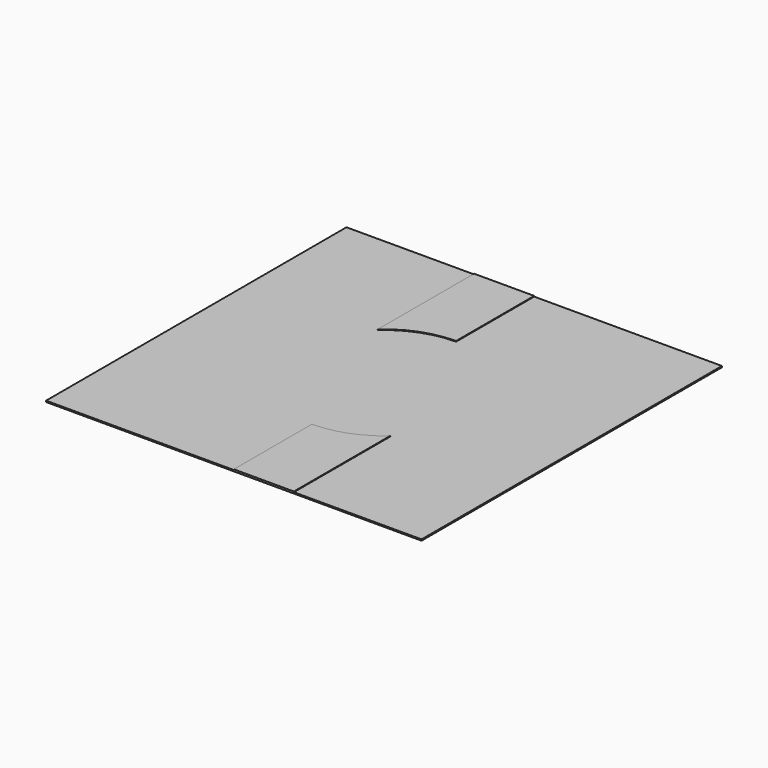
from build123d import *

# Parameters (mm, degrees)
F0_R     = 1790.7
F1_DEPTH = 25.4
F3_DEPTH = 25.4
F4_DEPTH = 25.4
F5_DEPTH = 38.1


# Not quite as in the source:
# - the program builds the solid bodies; features that only make, move or delete a surface that nothing else refers to are left out


with BuildPart() as f1:
    # F0 (on Top) → F1 (new body)
    with BuildSketch(Plane.XY):
        with BuildLine():
            Line((-1219.2, 3810.0001542995), (-3809.5957711624, 3810.0001542995))
            Line((-3809.5957711624, 3810.0001542995), (-3809.5957711624, -3809.9998457005))
            Line((-3809.5957711624, -3809.9998457005), (3.7253e-06, -3809.9998457005))
            Line((3.7253e-06, -3809.9998457005), (3.0473e-06, -3116.5800094754))
            Line((3.0473e-06, -3116.5800094754), (2.2873e-06, -2339.3399715424))
            Line((2.2873e-06, -2339.3399715424), (1.7881e-06, -1828.8))
            ThreePointArc((1.7881e-06, -1828.8), (-1708.414409752, -652.5562386122), (-1219.2, 1363.1070390839))
            Line((-1219.2, 1363.1070390839), (-1219.2, 2247.9000093898))
            Line((-1219.2, 2247.9000093898), (-1219.2, 3040.3800010681))
            Line((-1219.2, 3040.3800010681), (-1219.2, 3810.0001542995))
        make_face()
        with BuildLine():
            Line((3809.595778613, 3810.0001542995), (3.7253e-06, 3810.0001542995))
            Line((3.7253e-06, 3810.0001542995), (0, 3040.3800010681))
            Line((0, 3040.3800010681), (0, 2247.9000081977))
            Line((0, 2247.9000081977), (0, 1828.8))
            ThreePointArc((0, 1828.8), (1293.156881434, 1293.156881434), (1828.8, 0))
            ThreePointArc((1828.8, 0), (1669.4583559266, -746.6044721449), (1219.2000023767, -1363.1070369581))
            Line((1219.2000023767, -1363.1070369581), (1219.2000023767, -2339.3399703503))
            Line((1219.2000023767, -2339.3399703503), (1219.2000023767, -3116.5800082833))
            Line((1219.2000023767, -3116.5800082833), (1219.2000023767, -3809.9998457005))
            Line((1219.2000023767, -3809.9998457005), (3809.595778613, -3809.9998457005))
            Line((3809.595778613, -3809.9998457005), (3809.595778613, 3810.0001542995))
        make_face()
        with BuildLine():
            ThreePointArc((0, 1828.8), (-652.556237777, 1708.414410071), (-1219.2, 1363.1070390839))
            ThreePointArc((-1219.2, 1363.1070390839), (-1708.414409752, -652.5562386122), (1.7881e-06, -1828.8))
            ThreePointArc((1.7881e-06, -1828.8), (652.5562401017, -1708.4144091831), (1219.2000023767, -1363.1070369581))
            ThreePointArc((1219.2000023767, -1363.1070369581), (1669.4583559266, -746.6044721449), (1828.8, 0))
            ThreePointArc((1828.8, 0), (1293.156881434, 1293.156881434), (0, 1828.8))
        make_face()
        Circle(F0_R, mode=Mode.SUBTRACT)
    extrude(amount=F1_DEPTH)

    # F0 (on Top) → F3 (join)
    with BuildSketch(Plane.XY):
        with BuildLine():
            Line((-1219.2, 3810.0001542995), (-3809.5957711624, 3810.0001542995))
            Line((-3809.5957711624, 3810.0001542995), (-3809.5957711624, -3809.9998457005))
            Line((-3809.5957711624, -3809.9998457005), (3.7253e-06, -3809.9998457005))
            Line((3.7253e-06, -3809.9998457005), (3.0473e-06, -3116.5800094754))
            Line((3.0473e-06, -3116.5800094754), (2.2873e-06, -2339.3399715424))
            Line((2.2873e-06, -2339.3399715424), (1.7881e-06, -1828.8))
            ThreePointArc((1.7881e-06, -1828.8), (-1708.414409752, -652.5562386122), (-1219.2, 1363.1070390839))
            Line((-1219.2, 1363.1070390839), (-1219.2, 2247.9000093898))
            Line((-1219.2, 2247.9000093898), (-1219.2, 3040.3800010681))
            Line((-1219.2, 3040.3800010681), (-1219.2, 3810.0001542995))
        make_face()
        Polygon((3.7253e-06, 3810.0001542995), (-1219.2, 3810.0001542995), (-1219.2, 3040.3800010681), (0, 3040.3800010681), align=None)
        with BuildLine():
            Line((3809.595778613, 3810.0001542995), (3.7253e-06, 3810.0001542995))
            Line((3.7253e-06, 3810.0001542995), (0, 3040.3800010681))
            Line((0, 3040.3800010681), (0, 2247.9000081977))
            Line((0, 2247.9000081977), (0, 1828.8))
            ThreePointArc((0, 1828.8), (1293.156881434, 1293.156881434), (1828.8, 0))
            ThreePointArc((1828.8, 0), (1669.4583559266, -746.6044721449), (1219.2000023767, -1363.1070369581))
            Line((1219.2000023767, -1363.1070369581), (1219.2000023767, -2339.3399703503))
            Line((1219.2000023767, -2339.3399703503), (1219.2000023767, -3116.5800082833))
            Line((1219.2000023767, -3116.5800082833), (1219.2000023767, -3809.9998457005))
            Line((1219.2000023767, -3809.9998457005), (3809.595778613, -3809.9998457005))
            Line((3809.595778613, -3809.9998457005), (3809.595778613, 3810.0001542995))
        make_face()
        Polygon((3.0473e-06, -3116.5800094754), (3.7253e-06, -3809.9998457005), (1219.2000023767, -3809.9998457005), (1219.2000023767, -3116.5800082833), align=None)
    extrude(amount=F3_DEPTH)

    # F0 (on Top) → F4 (join)
    with BuildSketch(Plane.XY):
        Circle(F0_R)
    extrude(amount=F4_DEPTH)

    # F0 (on Top) → F5 (join)
    with BuildSketch(Plane.XY):
        Polygon((3.7253e-06, 3810.0001542995), (-1219.2, 3810.0001542995), (-1219.2, 3040.3800010681), (0, 3040.3800010681), align=None)
        with BuildLine():
            Line((0, 2247.9000081977), (-1219.2, 2247.9000093898))
            Line((-1219.2, 2247.9000093898), (-1219.2, 1363.1070390839))
            ThreePointArc((-1219.2, 1363.1070390839), (-652.556237777, 1708.414410071), (0, 1828.8))
            Line((0, 1828.8), (0, 2247.9000081977))
        make_face()
        Polygon((0, 3040.3800010681), (-1219.2, 3040.3800010681), (-1219.2, 2247.9000093898), (0, 2247.9000081977), align=None)
        with BuildLine():
            Line((1.7881e-06, -1828.8), (2.2873e-06, -2339.3399715424))
            Line((2.2873e-06, -2339.3399715424), (1219.2000023767, -2339.3399703503))
            Line((1219.2000023767, -2339.3399703503), (1219.2000023767, -1363.1070369581))
            ThreePointArc((1219.2000023767, -1363.1070369581), (652.5562401017, -1708.4144091831), (1.7881e-06, -1828.8))
        make_face()
        Polygon((2.2873e-06, -2339.3399715424), (3.0473e-06, -3116.5800094754), (1219.2000023767, -3116.5800082833), (1219.2000023767, -2339.3399703503), align=None)
        Polygon((3.0473e-06, -3116.5800094754), (3.7253e-06, -3809.9998457005), (1219.2000023767, -3809.9998457005), (1219.2000023767, -3116.5800082833), align=None)
    extrude(amount=F5_DEPTH)


solid = f1.part
